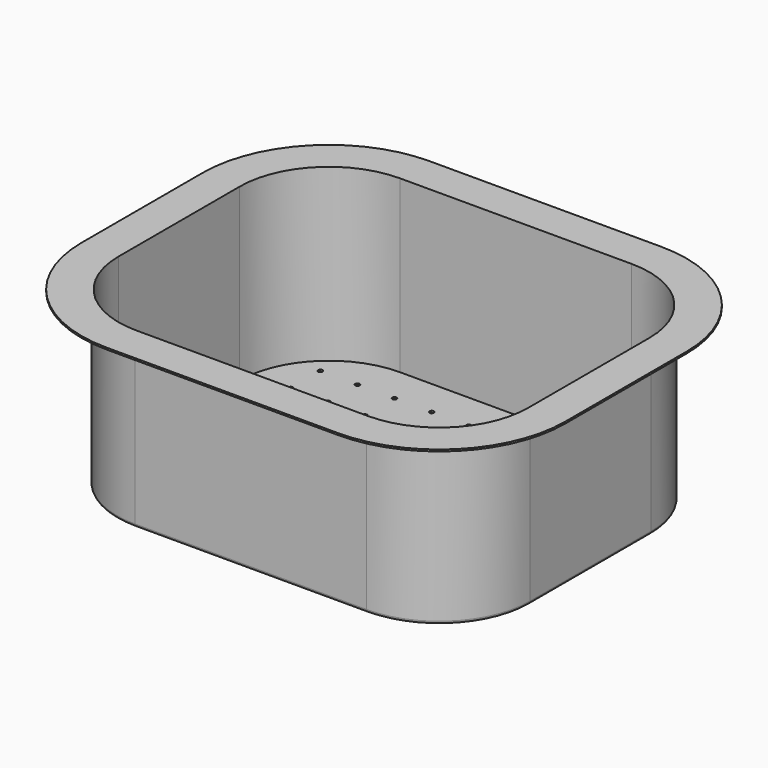
from build123d import *

# Parameters (mm, degrees)
F0_W     = 278.4
F0_H     = 224.4
F1_DEPTH = 57.5
F2_R     = 61.2
F3_T     = -1.2
F5_DEPTH = 1.2
F6_R     = 2
F7_R     = 1.5
F8_DEPTH = 1.2


# Not quite as in the source:
# - a feature names something its author has since deleted; it is built from what else it names


with BuildPart() as f1:
    # F0 (on Top) → F1 (new body, symmetric)
    with BuildSketch(Plane.XY):
        Rectangle(F0_W, F0_H)
    extrude(amount=F1_DEPTH, both=True)

    # F2
    f2_edges = [f1.edges().sort_by_distance(p)[0] for p in [
        (-139.2, -112.2, 0),
        (139.2, -112.2, 0),
        (139.2, 112.2, 0),
        (-139.2, 112.2, 0),
    ]]
    fillet(f2_edges, radius=F2_R)

    # F3
    f3_openings = [f1.faces().sort_by_distance(p)[0] for p in [
        (0, 0, 57.5),
    ]]
    offset(amount=F3_T, openings=f3_openings)

    # F4 (on face) → F5 (join)
    with BuildSketch(Plane.XY.offset(57.5)):
        with BuildLine():
            ThreePointArc((-163, -51), (-138.1040764009, -111.1040764009), (-78, -136))
            Line((-78, -136), (78, -136))
            ThreePointArc((78, -136), (138.1040764009, -111.1040764009), (163, -51))
            Line((163, -51), (163, 51))
            ThreePointArc((163, 51), (138.1040764009, 111.1040764009), (78, 136))
            Line((78, 136), (-78, 136))
            ThreePointArc((-78, 136), (-138.1040764009, 111.1040764009), (-163, 51))
            Line((-163, 51), (-163, -51))
        make_face()
        with BuildLine():
            ThreePointArc((138, -51), (120.4264068712, -93.4264068712), (78, -111))
            Line((78, -111), (-78, -111))
            ThreePointArc((-78, -111), (-120.4264068712, -93.4264068712), (-138, -51))
            Line((-138, -51), (-138, 51))
            ThreePointArc((-138, 51), (-120.4264068712, 93.4264068712), (-78, 111))
            Line((-78, 111), (78, 111))
            ThreePointArc((78, 111), (120.4264068712, 93.4264068712), (138, 51))
            Line((138, 51), (138, -51))
        make_face(mode=Mode.SUBTRACT)
    extrude(amount=F5_DEPTH)

    # F6
    f6_edges = [f1.edges().sort_by_distance(p)[0] for p in [
        (0, -112.2, -57.5),
        (139.2, 0, -57.5),
        (0, 112.2, -57.5),
        (-139.2, 0, -57.5),
        (-121.274935, -94.274935, -57.5),
        (-121.274935, 94.274935, -57.5),
        (121.274935, 94.274935, -57.5),
        (121.274935, -94.274935, -57.5),
    ]]
    fillet(f6_edges, radius=F6_R)

    # F7 (on face) → F8 (cut, through all)
    with BuildSketch(Plane.XY.offset(-56.3)):
        with Locations((-111.7, 86)):
            Circle(F7_R)
        with Locations((-111.7, 61)):
            Circle(F7_R)
        with Locations((-111.7, 36)):
            Circle(F7_R)
        with Locations((-111.7, 11)):
            Circle(F7_R)
        with Locations((-111.7, -14)):
            Circle(F7_R)
        with Locations((-111.7, -39)):
            Circle(F7_R)
        with Locations((-111.7, -64)):
            Circle(F7_R)
        with Locations((-111.7, -89)):
            Circle(F7_R)
        with Locations((-86.7, 86)):
            Circle(F7_R)
        with Locations((-86.7, 61)):
            Circle(F7_R)
        with Locations((-86.7, 36)):
            Circle(F7_R)
        with Locations((-86.7, 11)):
            Circle(F7_R)
        with Locations((-86.7, -14)):
            Circle(F7_R)
        with Locations((-86.7, -39)):
            Circle(F7_R)
        with Locations((-86.7, -64)):
            Circle(F7_R)
        with Locations((-86.7, -89)):
            Circle(F7_R)
        with Locations((-61.7, 86)):
            Circle(F7_R)
        with Locations((-61.7, 61)):
            Circle(F7_R)
        with Locations((-61.7, 36)):
            Circle(F7_R)
        with Locations((-61.7, 11)):
            Circle(F7_R)
        with Locations((-61.7, -14)):
            Circle(F7_R)
        with Locations((-61.7, -39)):
            Circle(F7_R)
        with Locations((-61.7, -64)):
            Circle(F7_R)
        with Locations((-61.7, -89)):
            Circle(F7_R)
        with Locations((-36.7, 86)):
            Circle(F7_R)
        with Locations((-36.7, 61)):
            Circle(F7_R)
        with Locations((-36.7, 36)):
            Circle(F7_R)
        with Locations((-36.7, 11)):
            Circle(F7_R)
        with Locations((-36.7, -14)):
            Circle(F7_R)
        with Locations((-36.7, -39)):
            Circle(F7_R)
        with Locations((-36.7, -64)):
            Circle(F7_R)
        with Locations((-36.7, -89)):
            Circle(F7_R)
        with Locations((-11.7, 86)):
            Circle(F7_R)
        with Locations((-11.7, 61)):
            Circle(F7_R)
        with Locations((-11.7, 36)):
            Circle(F7_R)
        with Locations((-11.7, 11)):
            Circle(F7_R)
        with Locations((-11.7, -14)):
            Circle(F7_R)
        with Locations((-11.7, -39)):
            Circle(F7_R)
        with Locations((-11.7, -64)):
            Circle(F7_R)
        with Locations((-11.7, -89)):
            Circle(F7_R)
        with Locations((13.3, 86)):
            Circle(F7_R)
        with Locations((13.3, 61)):
            Circle(F7_R)
        with Locations((13.3, 36)):
            Circle(F7_R)
        with Locations((13.3, 11)):
            Circle(F7_R)
        with Locations((13.3, -14)):
            Circle(F7_R)
        with Locations((13.3, -39)):
            Circle(F7_R)
        with Locations((13.3, -64)):
            Circle(F7_R)
        with Locations((13.3, -89)):
            Circle(F7_R)
        with Locations((38.3, 86)):
            Circle(F7_R)
        with Locations((38.3, 61)):
            Circle(F7_R)
        with Locations((38.3, 36)):
            Circle(F7_R)
        with Locations((38.3, 11)):
            Circle(F7_R)
        with Locations((38.3, -14)):
            Circle(F7_R)
        with Locations((38.3, -39)):
            Circle(F7_R)
        with Locations((38.3, -64)):
            Circle(F7_R)
        with Locations((38.3, -89)):
            Circle(F7_R)
        with Locations((63.3, 86)):
            Circle(F7_R)
        with Locations((63.3, 61)):
            Circle(F7_R)
        with Locations((63.3, 36)):
            Circle(F7_R)
        with Locations((63.3, 11)):
            Circle(F7_R)
        with Locations((63.3, -14)):
            Circle(F7_R)
        with Locations((63.3, -39)):
            Circle(F7_R)
        with Locations((63.3, -64)):
            Circle(F7_R)
        with Locations((63.3, -89)):
            Circle(F7_R)
        with Locations((88.3, 86)):
            Circle(F7_R)
        with Locations((88.3, 61)):
            Circle(F7_R)
        with Locations((88.3, 36)):
            Circle(F7_R)
        with Locations((88.3, 11)):
            Circle(F7_R)
        with Locations((88.3, -14)):
            Circle(F7_R)
        with Locations((88.3, -39)):
            Circle(F7_R)
        with Locations((88.3, -64)):
            Circle(F7_R)
        with Locations((88.3, -89)):
            Circle(F7_R)
        with Locations((113.3, 86)):
            Circle(F7_R)
        with Locations((113.3, 61)):
            Circle(F7_R)
        with Locations((113.3, 36)):
            Circle(F7_R)
        with Locations((113.3, 11)):
            Circle(F7_R)
        with Locations((113.3, -14)):
            Circle(F7_R)
        with Locations((113.3, -39)):
            Circle(F7_R)
        with Locations((113.3, -64)):
            Circle(F7_R)
        with Locations((113.3, -89)):
            Circle(F7_R)
    extrude(amount=-F8_DEPTH, mode=Mode.SUBTRACT)


solid = f1.part
